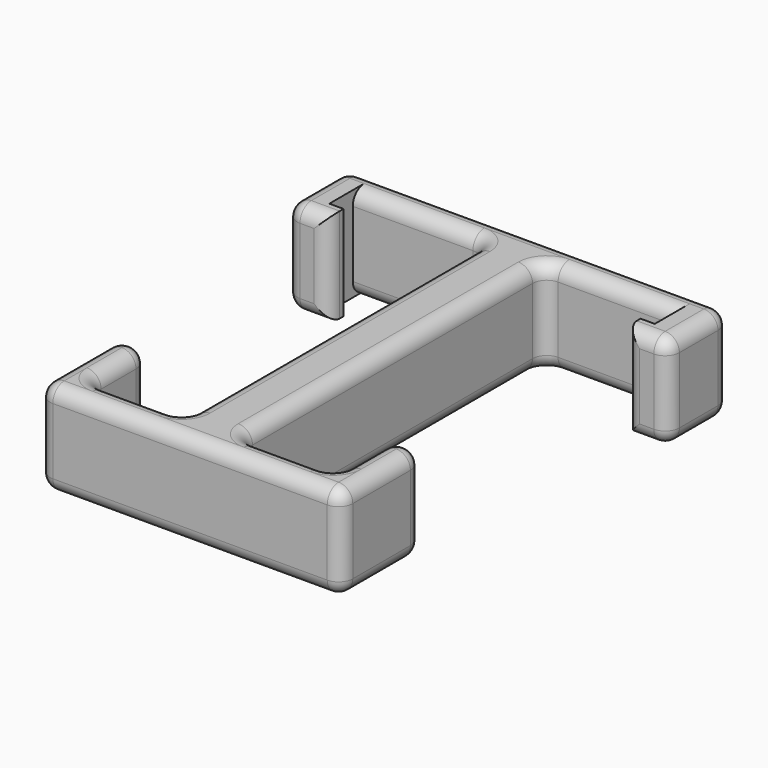
from build123d import *

# Parameters (mm, degrees)
F1_DEPTH = 10
F3_R     = 1.49999


# Not quite as in the source:
# - a fillet or chamfer is up to 0.001 mm smaller than in the source, because OpenCascade refuses the exact size
# - a feature names something its author has since deleted; it is built from what else it names


with BuildPart() as f1:
    # F0 (on Top) → F1 (new body)
    with BuildSketch(Plane.XY):
        Polygon((-15.7, 4.9212287627), (-17.2, 4.9212287627), (-17.2, 8.0212287627), (-3, 8.0212287627), (-3, -31.9787712373), (-13, -31.9787712373), (-13, -24.3669471227), (-16, -24.3669471227), (-16, -34.9787712373), (0, -34.9787712373), (0, 11.0212287627), (-20.2, 11.0212287627), (-20.2, 2.9212287627), (-15.7, 2.9212287627), align=None)
    extrude(amount=F1_DEPTH)

    # F2: F1 across face


with BuildPart() as f1_1:
    add(f1.part)
    add(f1.part.mirror(Plane(origin=(0, -11.9787712373, 5), x_dir=(0, 1, 0), z_dir=(1, 0, 0))))

    # F3 (radius 1.5 in the source; OpenCascade refuses exactly that, so slightly less here)
    f3_edges = [f1_1.edges().sort_by_distance(p)[0] for p in [
        (-3, -31.978771, 5),
        (-13, -31.978771, 5),
        (13, -31.978771, 5),
        (3, -31.978771, 5),
        (16, -34.978771, 5),
        (-16, -34.978771, 5),
        (0, 11.021229, 10),
        (0, 11.021229, 0),
        (0, -34.978771, 10),
        (0, -34.978771, 0),
        (3, -11.978771, 10),
        (-3, -11.978771, 10),
        (3, -11.978771, 0),
        (-3, -11.978771, 0),
        (-16, -29.672859, 10),
        (-16, -24.366947, 5),
        (-13, -28.172859, 0),
        (13, -24.366947, 5),
        (16, -29.672859, 0),
        (16, -29.672859, 10),
        (-13, -24.366947, 5),
        (-13, -28.172859, 10),
        (13, -28.172859, 0),
        (13, -28.172859, 10),
        (16, -24.366947, 5),
        (-8, -31.978771, 10),
        (8, -31.978771, 10),
        (-8, -31.978771, 0),
        (8, -31.978771, 0),
        (-14.5, -24.366947, 10),
        (-14.5, -24.366947, 0),
        (14.5, -24.366947, 10),
        (14.5, -24.366947, 0),
        (-16, -29.672859, 0),
        (-20.2, 6.971229, 10),
        (-20.2, 6.971229, 0),
        (20.2, 6.971229, 10),
        (20.2, 6.971229, 0),
        (3, 8.021229, 5),
        (-20.2, 2.921229, 5),
        (20.2, 2.921229, 5),
        (-15.7, 2.921229, 5),
        (15.7, 2.921229, 5),
        (-17.95, 2.921229, 10),
        (-17.95, 2.921229, 0),
        (17.95, 2.921229, 0),
        (17.95, 2.921229, 10),
        (-10.1, 8.021229, 10),
        (-10.1, 8.021229, 0),
        (10.1, 8.021229, 10),
        (10.1, 8.021229, 0),
        (-3, 8.021229, 5),
        (-20.2, 11.021229, 5),
        (20.2, 11.021229, 5),
    ]]
    fillet(f3_edges, radius=F3_R)


solid = f1_1.part
